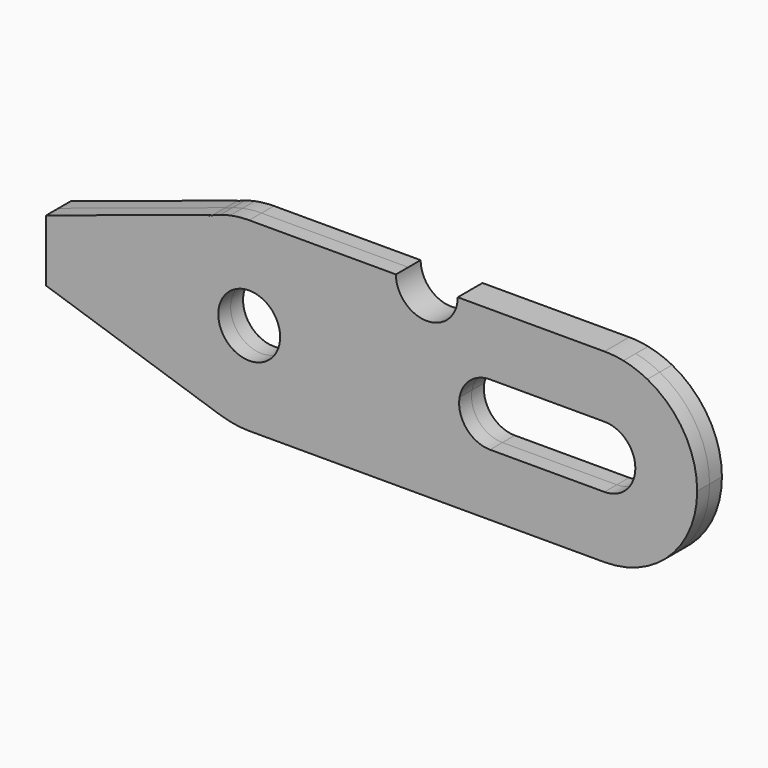
from build123d import *

# Parameters (mm, degrees)
F0_R     = 3.175
F1_DEPTH = 1.5875


with BuildPart() as f1:
    # F0 (on Front) → F1 (new body, symmetric)
    with BuildSketch(Plane.XZ):
        with BuildLine():
            Line((18.2378478348, 0), (3.175, 0))
            ThreePointArc((3.175, 0), (0, -3.175), (-3.175, 0))
            Line((-3.175, 0), (-18.2378478348, 0))
            ThreePointArc((-18.2378478348, 0), (-12.9826090881, -1.5809399099), (-9.4718777788, -5.7989573302))
            Line((-9.4718777788, -5.7989573302), (0, -10.7457929799))
            Line((0, -10.7457929799), (3.3629814094, -8.9894235763))
            ThreePointArc((3.3629814094, -8.9894235763), (4.4455137358, -7.0979565161), (6.4924834296, -6.35))
            Line((6.4924834296, -6.35), (8.4167772684, -6.35))
            Line((8.4167772684, -6.35), (9.4718777788, -5.7989573302))
            ThreePointArc((9.4718777788, -5.7989573302), (12.9826090881, -1.5809399099), (18.2378478348, 0))
        make_face()
        with BuildLine():
            ThreePointArc((20.1887122983, -0.2019236384), (19.2184911582, -0.0506153935), (18.2378478348, 0))
            ThreePointArc((18.2378478348, 0), (12.9826090881, -1.5809399099), (9.4718777788, -5.7989573302))
            Line((9.4718777788, -5.7989573302), (20.1887122983, -0.2019236384))
        make_face()
        with BuildLine():
            ThreePointArc((-9.4718777788, -5.7989573302), (-12.9826090881, -1.5809399099), (-18.2378478348, 0))
            ThreePointArc((-18.2378478348, 0), (-19.2184911582, -0.0506153935), (-20.1887122983, -0.2019236384))
            Line((-20.1887122983, -0.2019236384), (-9.4718777788, -5.7989573302))
        make_face()
        with BuildLine():
            ThreePointArc((22.6472823333, -1.082102843), (21.4483041232, -0.5573584248), (20.1887122983, -0.2019236384))
            Line((20.1887122983, -0.2019236384), (9.4718777788, -5.7989573302))
            ThreePointArc((9.4718777788, -5.7989573302), (9.3604581347, -6.0728156028), (9.2575917138, -6.35))
            Line((9.2575917138, -6.35), (18.2378478348, -6.35))
            ThreePointArc((18.2378478348, -6.35), (20.4829118651, -7.2799359697), (21.4128478348, -9.525))
            ThreePointArc((21.4128478348, -9.525), (20.4829118651, -11.7700640303), (18.2378478348, -12.7))
            Line((18.2378478348, -12.7), (9.2575917138, -12.7))
            ThreePointArc((9.2575917138, -12.7), (11.0435001343, -15.7673542165), (13.8284133364, -17.967897157))
            ThreePointArc((13.8284133364, -17.967897157), (15.9677124226, -18.7755194562), (18.2378478348, -19.05))
            ThreePointArc((18.2378478348, -19.05), (24.9730399256, -16.2601920908), (27.7628478348, -9.525))
            ThreePointArc((27.7628478348, -9.525), (26.384181016, -4.5891231072), (22.6472823333, -1.082102843))
        make_face()
        with BuildLine():
            ThreePointArc((9.2575917138, -6.35), (9.3604581347, -6.0728156028), (9.4718777788, -5.7989573302))
            Line((9.4718777788, -5.7989573302), (8.4167772684, -6.35))
            Line((8.4167772684, -6.35), (9.2575917138, -6.35))
        make_face()
        with BuildLine():
            Line((0, -10.7457929799), (-9.4718777788, -5.7989573302))
            ThreePointArc((-9.4718777788, -5.7989573302), (-8.9045341204, -7.6237161947), (-8.7128478348, -9.525))
            ThreePointArc((-8.7128478348, -9.525), (-10.0915146536, -14.4608768928), (-13.8284133364, -17.967897157))
            Line((-13.8284133364, -17.967897157), (0, -10.7457929799))
        make_face()
        with BuildLine():
            ThreePointArc((-8.7128478348, -9.525), (-8.9045341204, -7.6237161947), (-9.4718777788, -5.7989573302))
            Line((-9.4718777788, -5.7989573302), (-20.1887122983, -0.2019236384))
            ThreePointArc((-20.1887122983, -0.2019236384), (-20.7031117187, -0.3245598484), (-21.2099123798, -0.4755548601))
            ThreePointArc((-21.2099123798, -0.4755548601), (-21.9410366156, -0.7493508585), (-22.6472823333, -1.082102843))
            ThreePointArc((-22.6472823333, -1.082102843), (-27.7308527221, -10.3050533377), (-21.2099123798, -18.5744451399))
            ThreePointArc((-21.2099123798, -18.5744451399), (-19.7427830564, -18.9303599069), (-18.2378478348, -19.05))
            ThreePointArc((-18.2378478348, -19.05), (-15.9677124226, -18.7755194562), (-13.8284133364, -17.967897157))
            ThreePointArc((-13.8284133364, -17.967897157), (-10.0915146536, -14.4608768928), (-8.7128478348, -9.525))
        make_face()
        with Locations((-18.2378478348, -9.525)):
            Circle(F0_R, mode=Mode.SUBTRACT)
        with BuildLine():
            Line((13.8284133364, -17.967897157), (0, -10.7457929799))
            Line((0, -10.7457929799), (-13.8284133364, -17.967897157))
            ThreePointArc((-13.8284133364, -17.967897157), (-15.9677124226, -18.7755194562), (-18.2378478348, -19.05))
            Line((-18.2378478348, -19.05), (18.2378478348, -19.05))
            ThreePointArc((18.2378478348, -19.05), (15.9677124226, -18.7755194562), (13.8284133364, -17.967897157))
        make_face()
        with BuildLine():
            Line((3.3629814094, -8.9894235763), (0, -10.7457929799))
            Line((0, -10.7457929799), (13.8284133364, -17.967897157))
            ThreePointArc((13.8284133364, -17.967897157), (11.0435001343, -15.7673542165), (9.2575917138, -12.7))
            Line((9.2575917138, -12.7), (6.4924834296, -12.7))
            ThreePointArc((6.4924834296, -12.7), (4.0654399457, -11.5719696938), (3.3629814094, -8.9894235763))
        make_face()
        with BuildLine():
            Line((-22.6472823333, -1.082102843), (-21.9535177998, -0.7197735133))
            Line((-21.9535177998, -0.7197735133), (-39.097144814, -6.3501702098))
            Line((-39.097144814, -6.3501702098), (-39.097144814, -12.6998297902))
            Line((-39.097144814, -12.6998297902), (-21.2099123798, -18.5744451399))
            ThreePointArc((-21.2099123798, -18.5744451399), (-27.7308527221, -10.3050533377), (-22.6472823333, -1.082102843))
        make_face()
    extrude(amount=F1_DEPTH, both=True)


solid = f1.part
